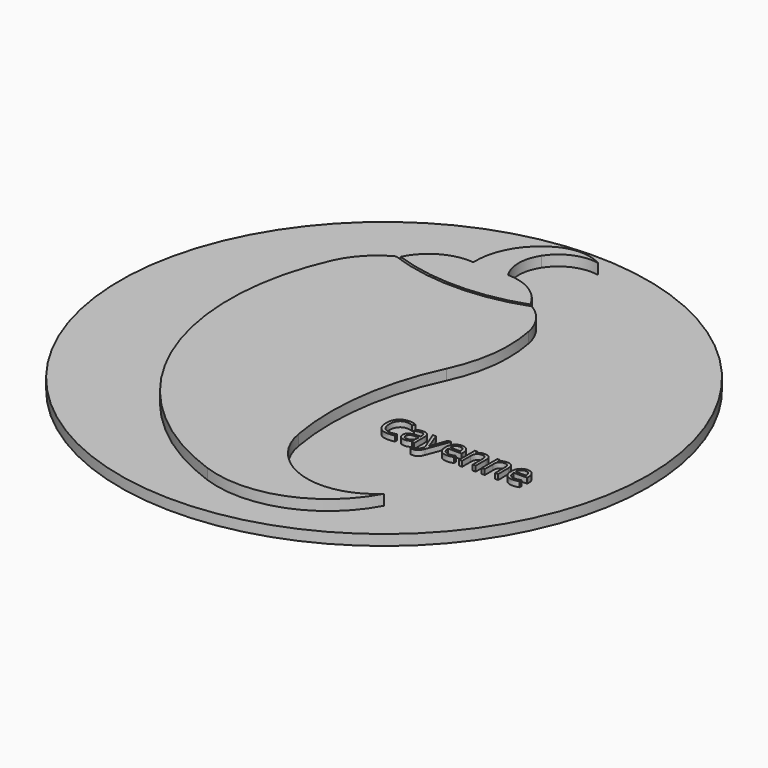
from build123d import *

# Parameters (mm, degrees)
F0_R         = 12.7
F1_DEPTH     = 0.508
F3_DEPTH     = 0.508
F5_DEPTH     = 0.508
F7_DEPTH     = 0.508
F8_TEXT_SIZE = 1.7638888889
F9_DEPTH     = 0.254


# Not quite as in the source:
# - Text() gives the source's letters only with a copy of the font that has no kerning and outlines rounded to 1/6400 em; it was checked with that copy


with BuildPart() as f1:
    # F0 (on Top) → F1 (new body)
    with BuildSketch(Plane.XY):
        Circle(F0_R)
    extrude(amount=F1_DEPTH)

    # F2 (on face) → F3 (join)
    with BuildSketch(Plane.XY.offset(0.508)):
        with BuildLine():
            ThreePointArc((-6.8939032355, 5.4748712447), (-6.9638355074, -4.0821123419), (0, -10.6277842571))
            ThreePointArc((0, -10.6277842571), (3.7105954478, -10.5808262174), (6.4925869183, -8.1249664713))
            ThreePointArc((6.4925869183, -8.1249664713), (3.1786973797, -8.8900199222), (0.9471852266, -6.3234026606))
            ThreePointArc((0.9471852266, -6.3234026606), (0.8663243967, -2.4307376781), (1.9685540187, 1.3034916936))
            ThreePointArc((1.9685540187, 1.3034916936), (2.5739515935, 3.3996371568), (2.4903307674, 5.579852647))
            ThreePointArc((2.4903307674, 5.579852647), (1.6096543537, 7.0448442334), (0, 7.62))
            Line((0, 7.62), (-4.064, 7.62))
            ThreePointArc((-4.064, 7.62), (-5.7545562324, 6.9110195745), (-6.8939032355, 5.4748712447))
        make_face()
    extrude(amount=F3_DEPTH)

    # F4 (on face) → F5 (join)
    with BuildSketch(Plane.XY.offset(1.016)):
        with BuildLine():
            ThreePointArc((-1.044166275, 11.5734093063), (-2.2597485424, 10.3603628917), (-2.6533177588, 8.6887693033))
            ThreePointArc((-2.6533177588, 8.6887693033), (-4.0740091472, 8.3853654003), (-5.0654162118, 7.3235132535))
            ThreePointArc((-5.0654162118, 7.3235132535), (-1.9497780392, 7.0385508074), (1.1645689099, 7.3372946759))
            ThreePointArc((1.1645689099, 7.3372946759), (0.2811255283, 8.317358048), (-0.9849906201, 8.6887693033))
            ThreePointArc((-0.9849906201, 8.6887693033), (-1.2837607801, 9.6978377551), (-0.9849906201, 10.7069062069))
            ThreePointArc((-0.9849906201, 10.7069062069), (-0.1099093619, 11.4451703345), (1.0277882677, 11.5734093063))
            ThreePointArc((1.0277882677, 11.5734093063), (-0.0081890037, 11.841665302), (-1.044166275, 11.5734093063))
        make_face()
    extrude(amount=-F5_DEPTH)

    # F6 (on face) → F7 (cut)
    with BuildSketch(Plane.XY.offset(1.016)):
        with BuildLine():
            ThreePointArc((1.1645689099, 7.3372946759), (-1.9492484598, 6.7991508831), (-5.0654162118, 7.3235132535))
            ThreePointArc((-5.0654162118, 7.3235132535), (-5.1457057191, 7.2855015459), (-5.2250551064, 7.2455644749))
            ThreePointArc((-5.2250551064, 7.2455644749), (-1.9559401597, 6.6721383217), (1.3114630436, 7.255238995))
            ThreePointArc((1.3114630436, 7.255238995), (1.2386956214, 7.2974835191), (1.1645689099, 7.3372946759))
        make_face()
    extrude(amount=-F7_DEPTH, mode=Mode.SUBTRACT)

    # F8 (on face) → F9 (join)
    with BuildSketch(Plane.XY.offset(0.508)):
        with Locations((2.54, -3.81)):
            Text('Cayenne', F8_TEXT_SIZE, font='Open Sans', text_align=(TextAlign.LEFT, TextAlign.BOTTOM))
    extrude(amount=F9_DEPTH)


solid = f1.part
